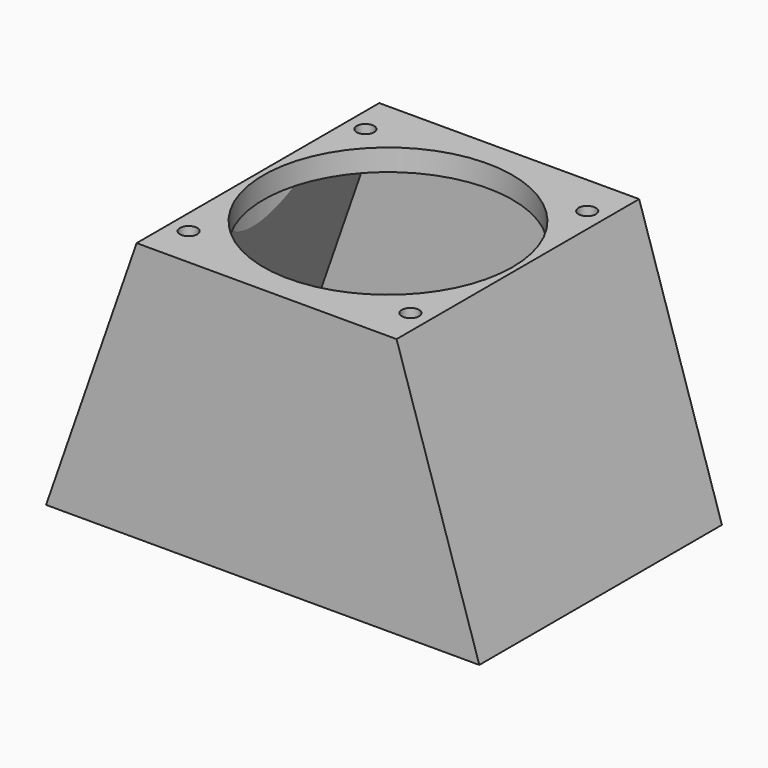
from build123d import *

# Parameters (mm, degrees)
F0_W      = 100
F0_H      = 70
F1_DEPTH  = 60
F3_DEPTH  = 70.001
F4_R      = 2
F5_DEPTH  = 60.001
F6_R      = 28.75
F7_DEPTH  = 60.001
F8_T      = -2.54
F9_R      = 31.29
F9_R_2    = 28.75
F9_R_3    = 4.54
F9_R_4    = 2
F10_DEPTH = 55
F11_W     = 8.9
F11_H     = 11
F12_DEPTH = 25.4


with BuildPart() as f1:
    # F0 (on Top) → F1 (new body)
    with BuildSketch(Plane.XY):
        Rectangle(F0_W, F0_H)
    extrude(amount=F1_DEPTH)

    # F2 (on face) → F3 (cut, through all)
    with BuildSketch(Plane.XZ.offset(35)):
        Polygon((-50, 60), (-50, 0), (-29.1, 60), align=None)
        Polygon((30.9, 60), (50, 0), (50, 60), align=None)
    extrude(amount=-F3_DEPTH, mode=Mode.SUBTRACT)

    # F4 (on face) → F5 (cut, through all)
    with BuildSketch(Plane.XY.offset(60)):
        with Locations((-24.7, 25.507)):
            Circle(F4_R)
        with Locations((26.5, 25.507)):
            Circle(F4_R)
        with Locations((26.5, -25.493)):
            Circle(F4_R)
        with Locations((-24.7, -25.493)):
            Circle(F4_R)
    extrude(amount=-F5_DEPTH, mode=Mode.SUBTRACT)

    # F6 (on face) → F7 (cut, through all)
    with BuildSketch(Plane.XY.offset(60)):
        with Locations((0.92, 0)):
            Circle(F6_R)
    extrude(amount=-F7_DEPTH, mode=Mode.SUBTRACT)

    # F8
    f8_openings = [f1.faces().sort_by_distance(p)[0] for p in [
        (0, 33.779344, 0),
    ]]
    offset(amount=F8_T, openings=f8_openings)

    # F9 (on face) → F10 (cut)
    with BuildSketch(Plane(origin=(0, 0, 0), x_dir=(1, 0, 0), z_dir=(0, 0, -1))):
        with Locations((0.92, 0)):
            Circle(F9_R)
        with Locations((0.92, 0)):
            Circle(F9_R_2, mode=Mode.SUBTRACT)
        with Locations((-24.7, 25.493)):
            Circle(F9_R_3)
        with Locations((-24.7, 25.493)):
            Circle(F9_R_4, mode=Mode.SUBTRACT)
        with Locations((26.5, 25.493)):
            Circle(F9_R_3)
        with Locations((26.5, 25.493)):
            Circle(F9_R_4, mode=Mode.SUBTRACT)
        with Locations((26.5, -25.507)):
            Circle(F9_R_3)
        with Locations((26.5, -25.507)):
            Circle(F9_R_4, mode=Mode.SUBTRACT)
        with Locations((-24.7, -25.507)):
            Circle(F9_R_3)
        with Locations((-24.7, -25.507)):
            Circle(F9_R_4, mode=Mode.SUBTRACT)
    extrude(amount=-F10_DEPTH, mode=Mode.SUBTRACT)

    # F11 (on face) → F12 (cut)
    with BuildSketch(Plane(origin=(0, 35, 0), x_dir=(-1, 0, 0), z_dir=(0, 1, 0))):
        with Locations((0.05, 5.5)):
            Rectangle(F11_W, F11_H)
    extrude(amount=-F12_DEPTH, mode=Mode.SUBTRACT)


solid = f1.part
